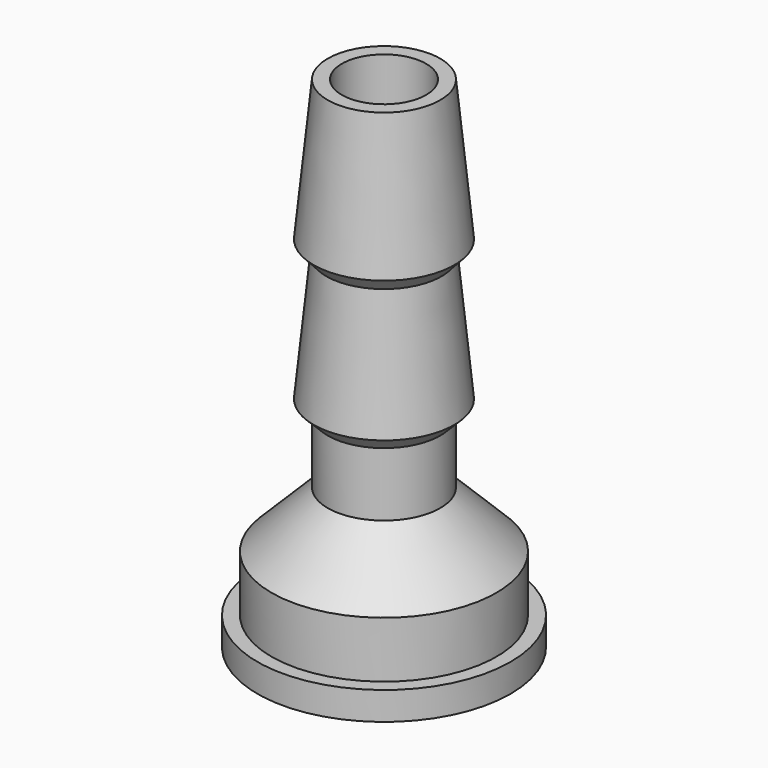
from build123d import *

# Parameters (mm, degrees)
F2_R        = 3
F3_DEPTH    = 35.5362252722
F4_T4_ANGLE = 180
F4_T6_ANGLE = 180


# Not quite as in the source:
# - a fillet or chamfer that OpenCascade refuses, or shapes differently, is made with other operations: its cross-section is extruded or revolved along the edge and cut away or added
# - a feature names something its author has since deleted; it is built from what else it names


with BuildPart() as f1:
    # F0 (on Front) → F1 (revolve)
    with BuildSketch(Plane.XZ):
        Polygon((-6, -5.5352252722), (0, 0.4647747278), (0, 25), (-4, 25), (-5, 15), (-4.099503719, 14.0049628098), (-5, 5), (-4, 4), (-4, -0.5352252722), (-8, -4.5352252722), (-8, -8.5352252722), (-9, -8.5352252722), (-9, -10.5352252722), (-6, -10.5352252722), align=None)
    revolve(axis=Axis((0, 0, 12.7323873639), (0, 0, 1)))

    # F2 (on face) → F3 (cut, through all)
    with BuildSketch(Plane.XY.offset(25)):
        Circle(F2_R)
    extrude(amount=-F3_DEPTH, mode=Mode.SUBTRACT)

    # F4: chamfer of 0.5 on 4 edges, made by hand

    # F4_s1 → F4_t2 (revolve)
    with BuildSketch(Plane.XZ):
        Polygon((-5.8535533906, -5.3887786628), (-6, -5.7423320534), (-6, -5.5352252722), align=None)
    revolve(axis=Axis((0, 0, -5.5352252722), (0, 0, 1)))

    # F4_s3 → F4_t4 (revolve, cut)
    with BuildSketch(Plane.XZ):
        Polygon((-3.1464466094, -2.6816718816), (-3, -2.328118491), (-3, -2.5352252722), align=None)
    revolve(axis=Axis((0, 0, -2.5352252722), (0, 0, 1)), revolution_arc=F4_T4_ANGLE, mode=Mode.SUBTRACT)

    # F4_s5 → F4_t6 (revolve, cut)
    with BuildSketch(Plane.XZ):
        Polygon((3.1464466094, -2.6816718816), (3, -2.328118491), (3, -2.5352252722), align=None)
    revolve(axis=Axis((0, 0, -2.5352252722), (0, 0, 1)), revolution_arc=F4_T6_ANGLE, mode=Mode.SUBTRACT)

    # F4_s7 → F4_t8 (revolve, cut)
    with BuildSketch(Plane.XZ):
        Polygon((-6, -10.0352252722), (-6.5, -10.5352252722), (-6, -10.5352252722), align=None)
    revolve(axis=Axis((0, 0, -10.5352252722), (0, 0, 1)), mode=Mode.SUBTRACT)


solid = f1.part
